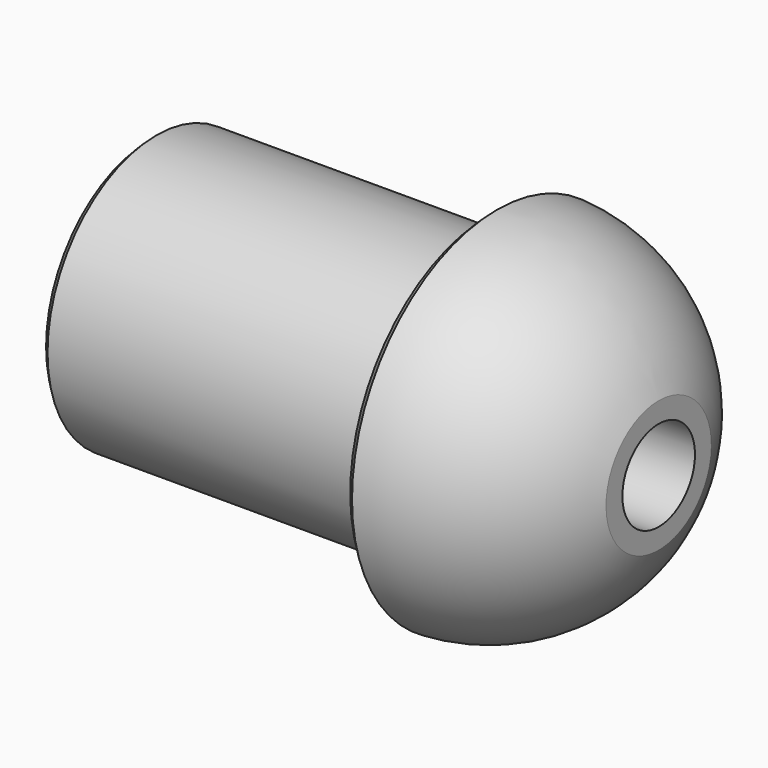
from build123d import *

# Parameters (mm, degrees)
F2_R      = 3.175
F3_DEPTH  = 15.24
F5_R      = 4.7625
F6_DEPTH  = 0.635
F7_R      = 6.35
F8_DEPTH  = 19.05
F10_R     = 1.0795
F11_DEPTH = 9.525


# Not quite as in the source:
# - a fillet or chamfer that OpenCascade refuses, or shapes differently, is made with other operations: its cross-section is extruded or revolved along the edge and cut away or added


with BuildPart() as f1:
    # F0 (on Front) → F1 (revolve)
    with BuildSketch(Plane.XZ):
        with BuildLine():
            Line((0, 9.525), (0, 0))
            Line((0, 0), (36.2827088845, 0))
            Line((36.2827088845, 0), (36.2827088845, 2.4049720118))
            ThreePointArc((36.2827088845, 2.4049720118), (31.8978835855, 9.7937006425), (23.8125, 12.7))
            Line((23.8125, 12.7), (23.8125, 9.525))
            Line((23.8125, 9.525), (0, 9.525))
        make_face()
    revolve(axis=Axis((18.1413544422, 0, 0), (-1, 0, 0)))

    # F2 (on face) → F3 (cut)
    with BuildSketch(Plane.YZ.offset(36.2827088845)):
        Circle(F2_R)
    extrude(amount=-F3_DEPTH, mode=Mode.SUBTRACT)

    # F5 (on offset) → F6 (cut)
    with BuildSketch(Plane.YZ.offset(36.2827088845)):
        Circle(F5_R)
    extrude(amount=-F6_DEPTH, mode=Mode.SUBTRACT)

    # F7 (on face) → F8 (cut)
    with BuildSketch(Plane(origin=(0, 0, 0), x_dir=(0, -1, 0), z_dir=(-1, 0, 0))):
        Circle(F7_R)
    extrude(amount=-F8_DEPTH, mode=Mode.SUBTRACT)

    # F9: chamfer of 0.508 on 2 edges, made by hand

    # F9_s1 → F9_t2 (revolve, cut)
    with BuildSketch(Plane.XZ):
        with BuildLine():
            Line((23.8125, 12.1814120692), (24.3416666667, 12.6889709054))
            ThreePointArc((24.3416666667, 12.6889709054), (24.0843208941, 12.6970907456), (23.8125, 12.7))
            Line((23.8125, 12.7), (23.8125, 12.1814120692))
        make_face()
    revolve(axis=Axis((23.8125, 0, 0), (-1, 0, 0)), mode=Mode.SUBTRACT)

    # F9_s3 → F9_t4 (revolve, cut)
    with BuildSketch(Plane.XZ):
        Polygon((0, 9.017), (0.508, 9.525), (0, 9.525), align=None)
    revolve(axis=Axis((0, 0, 0), (-1, 0, 0)), mode=Mode.SUBTRACT)

    # F10 (on face) → F11 (cut)
    with BuildSketch(Plane(origin=(0, 0, 0), x_dir=(0, -1, 0), z_dir=(-1, 0, 0))):
        with Locations((0, 7.9375)):
            Circle(F10_R)
        with Locations((0, -7.9375)):
            Circle(F10_R)
        with Locations((7.9375, 0)):
            Circle(F10_R)
        with Locations((-7.9375, 0)):
            Circle(F10_R)
    extrude(amount=-F11_DEPTH, mode=Mode.SUBTRACT)


solid = f1.part
